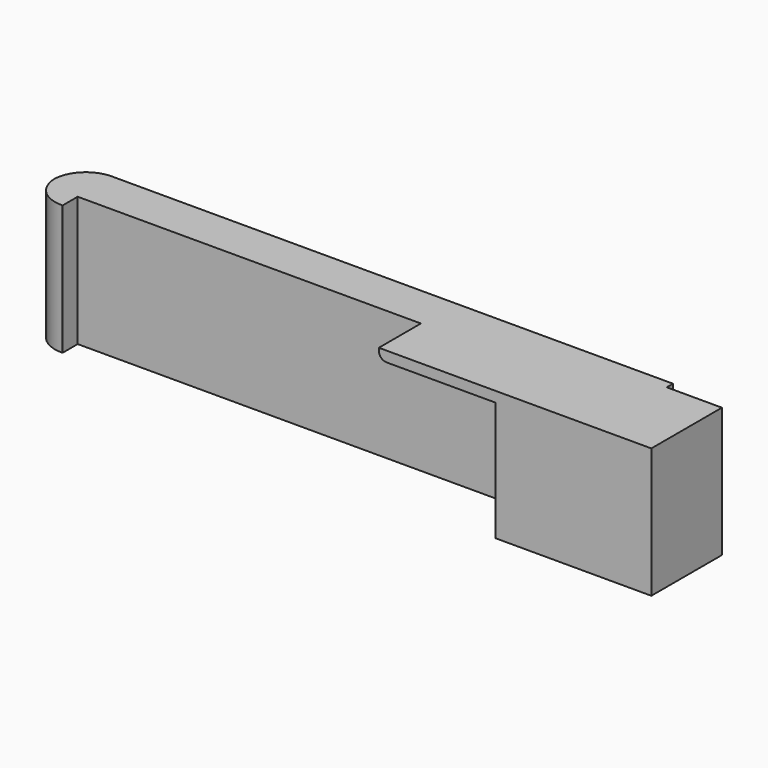
from build123d import *

# Parameters (mm, degrees)
F1_DEPTH    = 20
F2_W        = 18
F2_H        = 1.6
F3_DEPTH    = 8.1
F4_R        = 1.2
F5_T1_DEPTH = 29.1153030611
F5_T3_DEPTH = 31.6404483572
F5_T5_DEPTH = 45


# Not quite as in the source:
# - a fillet or chamfer that OpenCascade refuses, or shapes differently, is made with other operations: its cross-section is extruded or revolved along the edge and cut away or added


with BuildPart() as f1:
    # F0 (on Top) → F1 (new body)
    with BuildSketch(Plane.XY):
        Polygon((-24, 0.2), (-8.5, 0.2), (0, 0.2), (0, 1.7), (0, 13.8), (-8.5, 13.8), (-8.5, 15), (-100, 15), (-100, 8), (-96.9, 5.3927982226), (-94.9, 5.3927982226), (-94.9, 8.3), (-24, 8.3), align=None)
    extrude(amount=F1_DEPTH)

    # F2 (on face) → F3 (join)
    with BuildSketch(Plane.XZ.offset(-8.3)):
        with Locations((-33, 19.2)):
            Rectangle(F2_W, F2_H)
    extrude(amount=F3_DEPTH)

    # F4
    f4_edges = [f1.edges().sort_by_distance(p)[0] for p in [
        (-42, 4.25, 18.4),
    ]]
    fillet(f4_edges, radius=F4_R)

    # F5: fillet of radius 5 on 3 edges, made by hand

    # F5_s2 → F5_t1 (cut)
    with BuildSketch(Plane.XY.offset(-4.5576515305)):
        with BuildLine():
            ThreePointArc((-98.2952164267, 6.5662210444), (-96.7897023762, 5.6953049607), (-95.0769393878, 5.3927982226))
            Line((-95.0769393878, 5.3927982226), (-96.9, 5.3927982226))
            Line((-96.9, 5.3927982226), (-98.2952164267, 6.5662210444))
        make_face()
    extrude(amount=F5_T1_DEPTH, mode=Mode.SUBTRACT)

    # F5_s4 → F5_t3 (cut)
    with BuildSketch(Plane.XY.offset(-5.8202241786)):
        with BuildLine():
            ThreePointArc((-100, 10.3280896714), (-99.5327356637, 8.217566655), (-98.2182770389, 6.5015124932))
            Line((-98.2182770389, 6.5015124932), (-100, 8))
            Line((-100, 8), (-100, 10.3280896714))
        make_face()
    extrude(amount=F5_T3_DEPTH, mode=Mode.SUBTRACT)

    # F5_s6 → F5_t5 (cut)
    with BuildSketch(Plane.XY.offset(-12.5)):
        with BuildLine():
            ThreePointArc((-95, 15), (-98.5355339059, 13.5355339059), (-100, 10))
            Line((-100, 10), (-100, 15))
            Line((-100, 15), (-95, 15))
        make_face()
    extrude(amount=F5_T5_DEPTH, mode=Mode.SUBTRACT)


solid = f1.part
